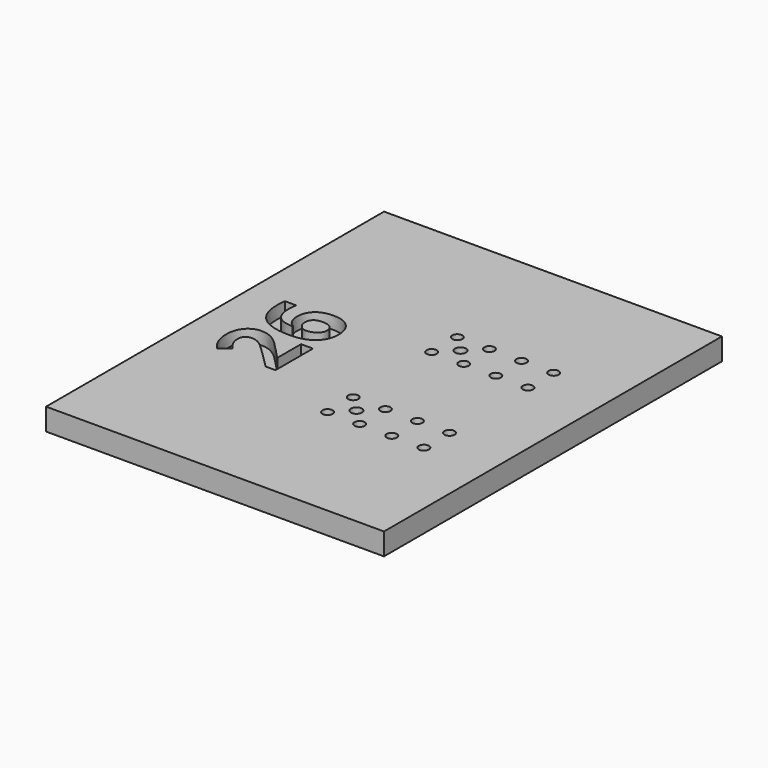
from build123d import *

# Parameters (mm, degrees)
F0_W         = 40
F0_H         = 50
F1_DEPTH     = 2.6
F2_TEXT_SIZE = 11.1111111111
F3_DEPTH     = 1.5
F4_R         = 0.6
F4_R_2       = 0.65
F5_DEPTH     = 2.6


# Not quite as in the source:
# - Text() gives the source's letters only with a copy of the font that has no kerning and outlines rounded to 1/6400 em; it was checked with that copy


with BuildPart() as f1:
    # F0 (on Top) → F1 (new body)
    with BuildSketch(Plane.XY):
        with Locations((-23.1587231159, 3.3350909071)):
            Rectangle(F0_W, F0_H)
    extrude(amount=F1_DEPTH)

    # F2 (on face) → F3 (cut)
    with BuildSketch(Plane.XY.offset(2.6)):
        with Locations(Location((-31.1587231159, -3.1649090929), (0, 0, 90))):
            Text('26', F2_TEXT_SIZE, font='Open Sans', font_style=FontStyle.BOLD, text_align=(TextAlign.LEFT, TextAlign.BOTTOM))
    extrude(amount=-F3_DEPTH, mode=Mode.SUBTRACT)

    # F4 (on face) → F5 (cut, through all)
    with BuildSketch(Plane.XY.offset(2.6)):
        with Locations((-22.1587231159, -2.4649090929)):
            Circle(F4_R)
        with Locations((-18.3587231159, -2.4649090929)):
            Circle(F4_R)
        with Locations((-14.5587231159, -2.4649090929)):
            Circle(F4_R)
        with Locations((-10.7587231159, -2.4649090929)):
            Circle(F4_R)
        with Locations((-22.1587231159, -6.2649090929)):
            Circle(F4_R)
        with Locations((-18.3587231159, -6.2649090929)):
            Circle(F4_R)
        with Locations((-14.5587231159, -6.2649090929)):
            Circle(F4_R)
        with Locations((-10.7587231159, -6.2649090929)):
            Circle(F4_R)
        with Locations((-20.2587231159, -4.3649090929)):
            Circle(F4_R_2)
        with Locations((-22.1587231159, 12.9350909071)):
            Circle(F4_R)
        with Locations((-18.3587231159, 12.9350909071)):
            Circle(F4_R)
        with Locations((-14.5587231159, 12.9350909071)):
            Circle(F4_R)
        with Locations((-10.7587231159, 12.9350909071)):
            Circle(F4_R)
        with Locations((-22.1587231159, 9.1350909071)):
            Circle(F4_R)
        with Locations((-18.3587231159, 9.1350909071)):
            Circle(F4_R)
        with Locations((-14.5587231159, 9.1350909071)):
            Circle(F4_R)
        with Locations((-10.7587231159, 9.1350909071)):
            Circle(F4_R)
        with Locations((-20.2587231159, 11.0350909071)):
            Circle(F4_R_2)
    extrude(amount=-F5_DEPTH, mode=Mode.SUBTRACT)


solid = f1.part
